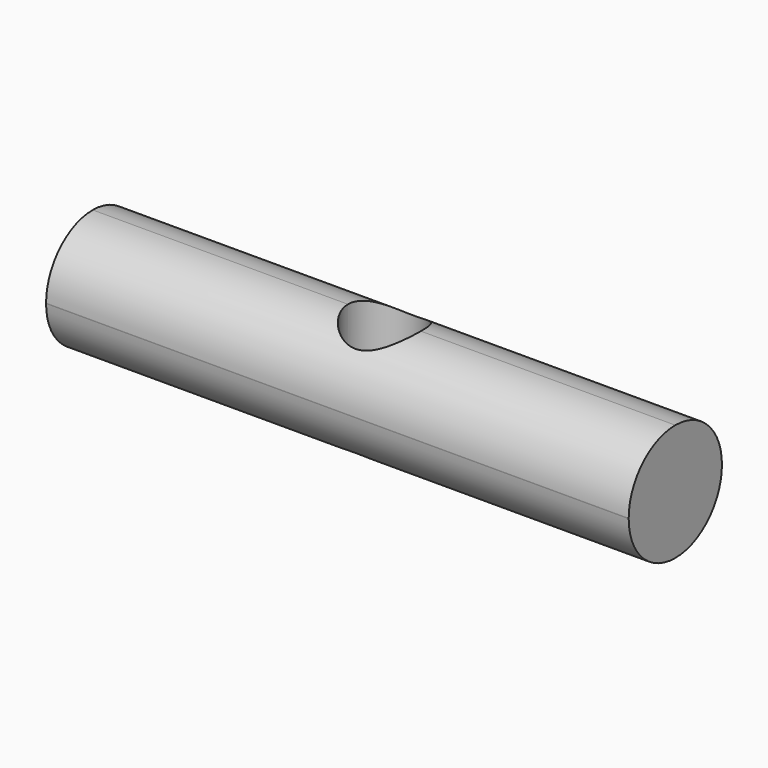
from build123d import *

# Parameters (mm, degrees)
F1_DEPTH    = 10.16
F3_D        = 6.35
F4_T1_DEPTH = 76.2


# Not quite as in the source:
# - a fillet or chamfer that OpenCascade refuses, or shapes differently, is made with other operations: its cross-section is extruded or revolved along the edge and cut away or added


with BuildPart() as f1:
    # F0 (on Front) → F1 (new body)
    with BuildSketch(Plane.XZ):
        Polygon((-25.4, 0), (0, 0), (25.4, 0), (25.4, 10.1957246661), (0, 10.1957246661), (-25.4, 10.1957246661), align=None)
    extrude(amount=F1_DEPTH)

    # F3 (through all)
    with Locations(Plane(origin=(0, 0, 0), x_dir=(1, 0, 0), z_dir=(0, 0, -1))):
        with Locations((0.0320593305, 5.0682155415)):
            Hole(F3_D / 2)

    # F4: fillet of radius 5.08 on 4 edges, made by hand

    # F4_s2 → F4_t1 (cut)
    with BuildSketch(Plane.YZ.offset(-38.1)):
        with BuildLine():
            ThreePointArc((-10.16, 5.1157246661), (-8.6721024484, 8.7078271145), (-5.08, 10.1957246661))
            Line((-5.08, 10.1957246661), (-10.16, 10.1957246661))
            Line((-10.16, 10.1957246661), (-10.16, 5.1157246661))
        make_face()
        with BuildLine():
            ThreePointArc((0, 5.1157246661), (-1.4878975516, 8.7078271145), (-5.08, 10.1957246661))
            Line((-5.08, 10.1957246661), (0, 10.1957246661))
            Line((0, 10.1957246661), (0, 5.1157246661))
        make_face()
        with BuildLine():
            ThreePointArc((-5.08, 0), (-8.6721024484, 1.4878975516), (-10.16, 5.08))
            Line((-10.16, 5.08), (-10.16, 0))
            Line((-10.16, 0), (-5.08, 0))
        make_face()
        with BuildLine():
            ThreePointArc((-5.08, 0), (-1.4878975516, 1.4878975516), (0, 5.08))
            Line((0, 5.08), (0, 0))
            Line((0, 0), (-5.08, 0))
        make_face()
    extrude(amount=F4_T1_DEPTH, mode=Mode.SUBTRACT)


solid = f1.part
